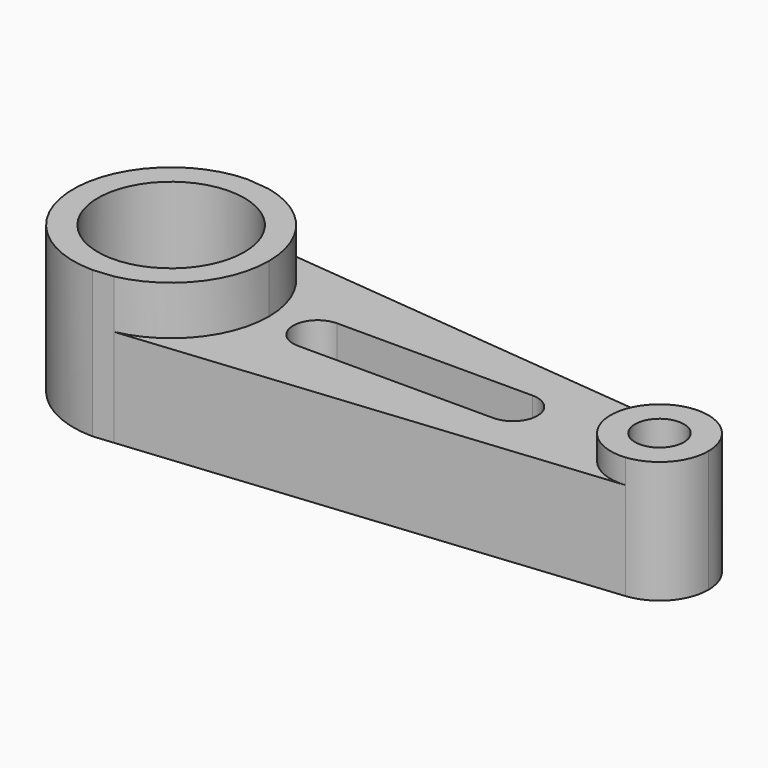
from build123d import *

# Parameters (mm, degrees)
F1_DEPTH = 25.4
F0_R     = 19.05
F2_DEPTH = 38.1
F0_R_2   = 6.35
F3_DEPTH = 31.75


# Not quite as in the source:
# - ends of sketch curves that miss each other by under 0.0002 mm in the source are joined


with BuildPart() as f1:
    # F0 (on Top) → F1 (new body)
    with BuildSketch(Plane.XY):
        with BuildLine():
            ThreePointArc((65.2491888918, -12.6376637775), (51.2924257238, -0.0024352029), (65.2443422993, 12.6381448126))
            Line((65.2443422993, 12.6381448126), (-57.5108169593, 24.798097839))
            ThreePointArc((-57.5108169593, 24.798097839), (-43.1987678598, 15.8987791704), (-37.6075745096, 0))
            ThreePointArc((-37.6075745096, 0), (-43.3336450312, -16.0653820023), (-57.9301334765, -24.8873379966))
            Line((-57.9301334765, -24.8873379966), (65.2491888918, -12.6376637775))
        make_face()
        with BuildLine():
            ThreePointArc((-24.9075745096, -6.35), (-31.2575745096, 0), (-24.9075745096, 6.35))
            Line((-24.9075745096, 6.35), (25.8924254904, 6.35))
            ThreePointArc((25.8924254904, 6.35), (32.2424254904, 0), (25.8924254904, -6.35))
            Line((25.8924254904, -6.35), (-24.9075745096, -6.35))
        make_face(mode=Mode.SUBTRACT)
    extrude(amount=F1_DEPTH)

    # F0 (on Top) → F2 (join)
    with BuildSketch(Plane.XY):
        with BuildLine():
            ThreePointArc((-37.6075745096, 0), (-43.1987678598, 15.8987791704), (-57.5108169593, 24.798097839))
            Line((-57.5108169593, 24.798097839), (-63.5323162428, 25.3945790694))
            ThreePointArc((-63.5323162428, 25.3945790694), (-88.4065859428, -0.2240942145), (-63.0841592169, -25.3998845427))
            Line((-63.0841592169, -25.3998845427), (-57.9301334765, -24.8873379966))
            ThreePointArc((-57.9301334765, -24.8873379966), (-43.3336450312, -16.0653820023), (-37.6075745096, 0))
        make_face()
        with Locations((-63.0075745096, 0)):
            Circle(F0_R, mode=Mode.SUBTRACT)
    extrude(amount=F2_DEPTH)

    # F0 (on Top) → F3 (join)
    with BuildSketch(Plane.XY):
        with BuildLine():
            ThreePointArc((65.2491888918, -12.6376637775), (73.406534455, -8.524350556), (76.6924254904, 0))
            ThreePointArc((76.6924254904, 0), (73.4048997526, 8.5261555383), (65.2443422993, 12.6381448126))
            ThreePointArc((65.2443422993, 12.6381448126), (51.2924257238, -0.0024352029), (65.2491888918, -12.6376637775))
        make_face()
        with Locations((63.9924254904, 0)):
            Circle(F0_R_2, mode=Mode.SUBTRACT)
    extrude(amount=F3_DEPTH)


solid = f1.part
